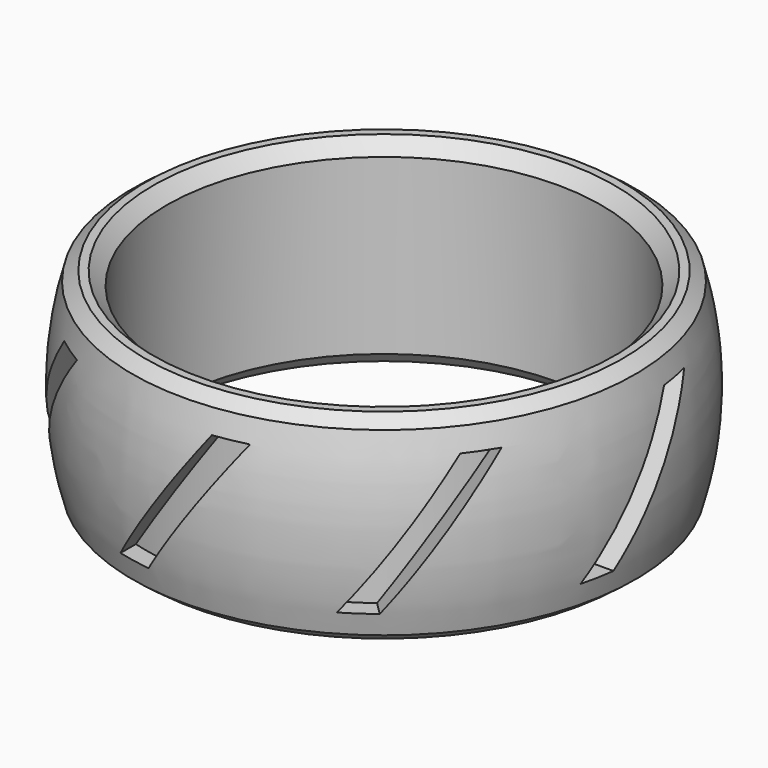
from build123d import *

# Parameters (mm, degrees)
F4_DEPTH        = 25
F4_COPIES_COUNT = 8
F5_R            = 11.5
F5_R_2          = 10.5
F6_DEPTH        = 4.825


# Not quite as in the source:
# - a fillet or chamfer that OpenCascade refuses, or shapes differently, is made with other operations: its cross-section is extruded or revolved along the edge and cut away or added
# - a pattern or mirror of a feature is missing from the dataset's text; its kind, count and spacing are read off the source's solid


with BuildPart() as f2:
    # F1 (on Right) → F2 (revolve)
    with BuildSketch(Plane.YZ):
        with BuildLine():
            Line((10.5, 4.825), (10.5, 0))
            Line((10.5, 0), (10.5, -4.825))
            Line((10.5, -4.825), (12, -4.825))
            ThreePointArc((12, -4.825), (12.7448574245, 0), (12, 4.825))
            Line((12, 4.825), (10.5, 4.825))
        make_face()
    revolve(axis=Axis((0, 0, 1.3494491577), (0, 0, 1)))

    # F3 (on Front) → F4 (cut)
    with BuildSketch(Plane.XZ):
        Polygon((3.1281900645, -3.325), (-1.5281900645, 3.325), (-3.1281900645, 3.325), (1.5281900645, -3.325), align=None)
    f4 = extrude(amount=-F4_DEPTH, mode=Mode.SUBTRACT)

    # F4_copies: F4 ×8 about axis
    f4_copies_axis = Axis((0, 0, 0), (0, 0, 1))
    for i in range(1, F4_COPIES_COUNT):
        add(f4.rotate(f4_copies_axis, i * 360 / F4_COPIES_COUNT), mode=Mode.SUBTRACT)

    # F5 (on Top) → F6 (join, symmetric)
    with BuildSketch(Plane.XY):
        Circle(F5_R)
        Circle(F5_R_2, mode=Mode.SUBTRACT)
    extrude(amount=F6_DEPTH, both=True)

    # F7: chamfer of 0.637 on 4 edges, made by hand

    # F7_s1 → F7_t2 (revolve, cut)
    with BuildSketch(Plane.YZ):
        with BuildLine():
            Line((11.5056834123, 4.8403663307), (12.1592080907, 4.3462817849))
            Line((12.1592080907, 4.3462817849), (12.1714655836, 4.3497547472))
            ThreePointArc((12.1714655836, 4.3497547472), (12.0863452232, 4.5876567471), (12.0121469073, 4.8288419063))
            Line((12.0121469073, 4.8288419063), (12, 4.83774))
            ThreePointArc((12, 4.83774), (11.7528417061, 4.83774), (11.5056834123, 4.8531063307))
            Line((11.5056834123, 4.8531063307), (11.5056834123, 4.8403663307))
        make_face()
    revolve(axis=Axis((0, 0, 4.825), (0, 0, 1)), mode=Mode.SUBTRACT)

    # F7_s3 → F7_t4 (revolve, cut)
    with BuildSketch(Plane.YZ):
        with BuildLine():
            Line((11.5056834123, -4.8403663307), (12.1592080907, -4.3462817849))
            Line((12.1592080907, -4.3462817849), (12.1714655836, -4.3497547472))
            ThreePointArc((12.1714655836, -4.3497547472), (12.0863452232, -4.5876567471), (12.0121469073, -4.8288419063))
            Line((12.0121469073, -4.8288419063), (12, -4.83774))
            ThreePointArc((12, -4.83774), (11.7528417061, -4.83774), (11.5056834123, -4.8531063307))
            Line((11.5056834123, -4.8531063307), (11.5056834123, -4.8403663307))
        make_face()
    revolve(axis=Axis((0, 0, -4.825), (0, 0, 1)), mode=Mode.SUBTRACT)

    # F7_s5 → F7_t6 (revolve, cut)
    with BuildSketch(Plane.YZ):
        with BuildLine():
            Line((11.1550170808, 4.8430170808), (10.4819829192, 4.1699829192))
            Line((10.4819829192, 4.1699829192), (10.4692429192, 4.1699829192))
            ThreePointArc((10.4692429192, 4.1699829192), (10.48726, 4.4974914596), (10.48726, 4.825))
            Line((10.48726, 4.825), (10.5, 4.83774))
            ThreePointArc((10.5, 4.83774), (10.8275085404, 4.83774), (11.1550170808, 4.8557570808))
            Line((11.1550170808, 4.8557570808), (11.1550170808, 4.8430170808))
        make_face()
    revolve(axis=Axis((0, 0, 4.825), (0, 0, -1)), mode=Mode.SUBTRACT)

    # F7_s7 → F7_t8 (revolve, cut)
    with BuildSketch(Plane.YZ):
        with BuildLine():
            Line((10.4819829192, -4.1699829192), (11.1550170808, -4.8430170808))
            Line((11.1550170808, -4.8430170808), (11.1550170808, -4.8557570808))
            ThreePointArc((11.1550170808, -4.8557570808), (10.8275085404, -4.83774), (10.5, -4.83774))
            Line((10.5, -4.83774), (10.48726, -4.825))
            ThreePointArc((10.48726, -4.825), (10.48726, -4.4974914596), (10.4692429192, -4.1699829192))
            Line((10.4692429192, -4.1699829192), (10.4819829192, -4.1699829192))
        make_face()
    revolve(axis=Axis((0, 0, -4.825), (0, 0, 1)), mode=Mode.SUBTRACT)


solid = f2.part
